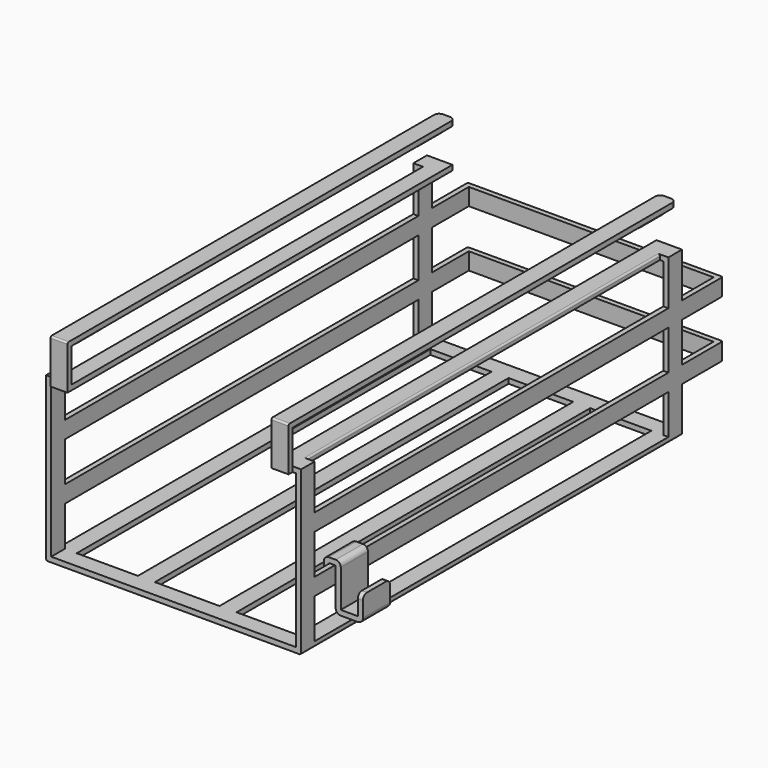
from build123d import *

# Parameters (mm, degrees)
F0_W           = 10
F0_H           = 260
F1_DEPTH       = 3
F2_W           = 3
F2_H           = 10
F3_DEPTH       = 90
F4_W           = 2
F4_H           = 10
F4_W_2         = 3
F4_W_3         = 10
F4_H_2         = 3
F4_W_4         = 5
F5_DEPTH       = 3
F6_W           = 10
F6_H           = 3
F7_DEPTH       = 20
F8_W           = 10
F8_H           = 282
F8_H_2         = 285
F8_H_3         = 3
F9_DEPTH       = 3
F10_W          = 3
F10_H          = 10
F11_DEPTH      = 30
F11_DEPTH_BACK = 270
F12_W          = 3
F12_H          = 10
F13_DEPTH      = 144
F14_R          = 1
F15_R          = 3
F17_DEPTH      = 1
F18_W          = 3
F18_H          = 20
F19_DEPTH      = 10
F18_W_2        = 0.5
F20_DEPTH      = 3
F21_DEPTH      = 25
F22_W          = 20
F22_H          = 3
F23_DEPTH      = 10
F24_W          = 3
F24_H          = 20
F25_DEPTH      = 15
F26_R          = 3


# Not quite as in the source:
# - a feature names something its author has since deleted; it is built from what else it names


with BuildPart() as f1:
    # F0 (on Top) → F1 (new body)
    with BuildSketch(Plane.XY):
        Polygon((-5.2808651924, 185.6500792865), (-155.2808651924, 185.6500792865), (-155.2808651924, 175.6500792865), (-145.2808651924, 175.6500792865), (-109.2808651924, 175.6500792865), (-99.2808651924, 175.6500792865), (-61.2808651924, 175.6500792865), (-51.2808651924, 175.6500792865), (-15.2808651924, 175.6500792865), (-5.2808651924, 175.6500792865), align=None)
        with Locations((-104.2808651924, 45.6500792865)):
            Rectangle(F0_W, F0_H)
        with Locations((-56.2808651924, 45.6500792865)):
            Rectangle(F0_W, F0_H)
        Polygon((-145.2808651924, -84.3499207135), (-155.2808651924, -84.3499207135), (-155.2808651924, -94.3499207135), (-5.2808651924, -94.3499207135), (-5.2808651924, -84.3499207135), (-15.2808651924, -84.3499207135), (-51.2808651924, -84.3499207135), (-61.2808651924, -84.3499207135), (-99.2808651924, -84.3499207135), (-109.2808651924, -84.3499207135), align=None)
        with Locations((-150.2808651924, 45.6500792865)):
            Rectangle(F0_W, F0_H)
        with Locations((-10.2808651924, 45.6500792865)):
            Rectangle(F0_W, F0_H)
    extrude(amount=F1_DEPTH)

    # F2 (on face) → F3 (join)
    with BuildSketch(Plane.XY.offset(3)):
        with Locations((-153.7808651924, 180.6500792865)):
            Rectangle(F2_W, F2_H)
        with Locations((-6.7808651924, 180.6500792865)):
            Rectangle(F2_W, F2_H)
        with Locations((-6.7808651924, -89.3499207135)):
            Rectangle(F2_W, F2_H)
        with Locations((-153.7808651924, -89.3499207135)):
            Rectangle(F2_W, F2_H)
    extrude(amount=F3_DEPTH)

    # F4 (on face) → F5 (join)
    with BuildSketch(Plane.XY.offset(93)):
        Polygon((-140.2808651924, 185.6500792865), (-150.2808651924, 185.6500792865), (-150.2808651924, 175.6500792865), (-150.2808651924, -84.3499207135), (-150.2808651924, -94.3499207135), (-140.2808651924, -94.3499207135), align=None)
        with Locations((-151.2808651924, 180.6500792865)):
            Rectangle(F4_W, F4_H)
        with Locations((-153.7808651924, 180.6500792865)):
            Rectangle(F4_W_2, F4_H)
        with Locations((-145.2808651924, -95.8499207135)):
            Rectangle(F4_W_3, F4_H_2)
        with Locations((-15.2808651924, -95.8499207135)):
            Rectangle(F4_W_3, F4_H_2)
        Polygon((-10.2808651924, 185.6500792865), (-20.2808651924, 185.6500792865), (-20.2808651924, -94.3499207135), (-10.2808651924, -94.3499207135), (-10.2808651924, -84.3499207135), (-10.2808651924, 175.6500792865), align=None)
        with Locations((-7.7808651924, -89.3499207135)):
            Rectangle(F4_W_4, F4_H)
        with Locations((-7.7808651924, 180.6500792865)):
            Rectangle(F4_W_4, F4_H)
        with Locations((-152.7808651924, -89.3499207135)):
            Rectangle(F4_W_4, F4_H)
    extrude(amount=F5_DEPTH)

    # F6 (on face) → F7 (join)
    with BuildSketch(Plane.XY.offset(96)):
        with Locations((-145.2808651924, -95.8499207135)):
            Rectangle(F6_W, F6_H)
        with Locations((-15.2808651924, -95.8499207135)):
            Rectangle(F6_W, F6_H)
    extrude(amount=F7_DEPTH)

    # F8 (on face) → F9 (join)
    with BuildSketch(Plane.XY.offset(116)):
        with Locations((-145.2808651924, 46.6500792865)):
            Rectangle(F8_W, F8_H)
        with Locations((-15.2808651924, 45.1500792865)):
            Rectangle(F8_W, F8_H_2)
        with Locations((-145.2808651924, -95.8499207135)):
            Rectangle(F8_W, F8_H_3)
    extrude(amount=F9_DEPTH)

    # F10 (on face) → F11 (join, two sides)
    with BuildSketch(Plane(origin=(0, 185.6500792865, 0), x_dir=(-1, 0, 0), z_dir=(0, 1, 0))) as f11_sk:
        with Locations((153.7808651924, 64.6666666667)):
            Rectangle(F10_W, F10_H)
        with Locations((153.7808651924, 31.3333333333)):
            Rectangle(F10_W, F10_H)
        with Locations((6.7808651924, 64.6666666667)):
            Rectangle(F10_W, F10_H)
        with Locations((6.7808651924, 31.3333333333)):
            Rectangle(F10_W, F10_H)
    extrude(amount=F11_DEPTH)
    extrude(f11_sk.sketch, amount=-F11_DEPTH_BACK)

    # F12 (on face) → F13 (join, through all)
    with BuildSketch(Plane.YZ.offset(-152.2808651924)):
        with Locations((214.1500792864, 64.6666666667)):
            Rectangle(F12_W, F12_H)
        with Locations((214.1500792864, 31.3333333333)):
            Rectangle(F12_W, F12_H)
    extrude(amount=F13_DEPTH)

    # F14
    f14_edges = [f1.edges().sort_by_distance(p)[0] for p in [
        (-155.280865, 45.650079, 0),
        (-5.280865, 45.650079, 0),
        (-5.280865, 215.650079, 31.333333),
        (-5.280865, 215.650079, 64.666667),
        (-155.280865, 215.650079, 64.666667),
        (-155.280865, 215.650079, 31.333333),
        (-150.280865, 45.650079, 96),
        (-145.280865, -97.349921, 119),
        (-15.280865, -97.349921, 119),
        (-10.280865, 45.650079, 96),
    ]]
    fillet(f14_edges, radius=F14_R)

    # F15
    f15_edges = [f1.edges().sort_by_distance(p)[0] for p in [
        (-140.280865, 187.650079, 117.5),
        (-150.280865, 187.650079, 117.5),
        (-20.280865, 187.650079, 117.5),
        (-10.280865, 187.650079, 117.5),
    ]]
    fillet(f15_edges, radius=F15_R)


with BuildPart() as f17:
    # F16 (on face) → F17 (new body)
    with BuildSketch(Plane(origin=(0, 0, 116), x_dir=(1, 0, 0), z_dir=(0, 0, -1))):
        with BuildLine():
            ThreePointArc((-149.3451507241, -179.0511412621), (-145.3451507241, -183.0511412621), (-141.3451507241, -179.0511412621))
            Line((-141.3451507241, -179.0511412621), (-141.3451507241, -162.0511412621))
            ThreePointArc((-141.3451507241, -162.0511412621), (-145.3451507241, -158.0511412621), (-149.3451507241, -162.0511412621))
            Line((-149.3451507241, -162.0511412621), (-149.3451507241, -179.0511412621))
        make_face()
    extrude(amount=F17_DEPTH)


with BuildPart() as f17b:
    # F16 (on face) → F17, piece 2 (new body)
    with BuildSketch(Plane(origin=(0, 0, 116), x_dir=(1, 0, 0), z_dir=(0, 0, -1))):
        with BuildLine():
            ThreePointArc((-11.2165796608, -162.0511412621), (-15.2165796608, -158.0511412621), (-19.2165796608, -162.0511412621))
            Line((-19.2165796608, -162.0511412621), (-19.2165796608, -179.0511412621))
            ThreePointArc((-19.2165796608, -179.0511412621), (-15.2165796608, -183.0511412621), (-11.2165796608, -179.0511412621))
            Line((-11.2165796608, -179.0511412621), (-11.2165796608, -162.0511412621))
        make_face()
    extrude(amount=F17_DEPTH)


with BuildPart() as f17c:
    # F16 (on face) → F17, piece 3 (new body)
    with BuildSketch(Plane(origin=(0, 0, 116), x_dir=(1, 0, 0), z_dir=(0, 0, -1))):
        with BuildLine():
            ThreePointArc((-11.2165796608, 88.7509826891), (-15.2165796608, 92.7509826891), (-19.2165796608, 88.7509826891))
            Line((-19.2165796608, 88.7509826891), (-19.2165796608, 71.7509826891))
            ThreePointArc((-19.2165796608, 71.7509826891), (-15.2165796608, 67.7509826891), (-11.2165796608, 71.7509826891))
            Line((-11.2165796608, 71.7509826891), (-11.2165796608, 88.7509826891))
        make_face()
    extrude(amount=F17_DEPTH)


with BuildPart() as f17d:
    # F16 (on face) → F17, piece 4 (new body)
    with BuildSketch(Plane(origin=(0, 0, 116), x_dir=(1, 0, 0), z_dir=(0, 0, -1))):
        with BuildLine():
            Line((-149.3451507241, 88.7509826891), (-149.3451507241, 71.7509826891))
            ThreePointArc((-149.3451507241, 71.7509826891), (-145.3451507241, 67.7509826891), (-141.3451507241, 71.7509826891))
            Line((-141.3451507241, 71.7509826891), (-141.3451507241, 88.7509826891))
            ThreePointArc((-141.3451507241, 88.7509826891), (-145.3451507241, 92.7509826891), (-149.3451507241, 88.7509826891))
        make_face()
    extrude(amount=F17_DEPTH)


with BuildPart() as f19:
    # F18 (on face) → F19 (new body, through all)
    with BuildSketch(Plane.XY.offset(36.3333333333)):
        with Locations((-10.2808651924, -59.5772841573)):
            Rectangle(F18_W, F18_H)
    extrude(amount=-F19_DEPTH)

    # F18 (on face) → F20 (join)
    with BuildSketch(Plane.XY.offset(36.3333333333)):
        with Locations((-10.2808651924, -59.5772841573)):
            Rectangle(F18_W, F18_H)
        with Locations((-6.7808651924, -59.5772841573)):
            Rectangle(F18_W, F18_H)
        with Locations((-8.5308651924, -59.5772841573)):
            Rectangle(F18_W_2, F18_H)
        with Locations((-5.0308651924, -59.5772841573)):
            Rectangle(F18_W_2, F18_H)
        with Locations((-3.2808651924, -59.5772841573)):
            Rectangle(F18_W, F18_H)
    extrude(amount=F20_DEPTH)

    # F18 (on face) → F21 (join)
    with BuildSketch(Plane.XY.offset(36.3333333333)):
        with Locations((-3.2808651924, -59.5772841573)):
            Rectangle(F18_W, F18_H)
    extrude(amount=-F21_DEPTH)

    # F22 (on face) → F23 (join)
    with BuildSketch(Plane.YZ.offset(-1.7808651924)):
        with Locations((-59.5772841573, 12.8333333333)):
            Rectangle(F22_W, F22_H)
    extrude(amount=F23_DEPTH)

    # F24 (on face) → F25 (join)
    with BuildSketch(Plane(origin=(0, 0, 11.3333333333), x_dir=(1, 0, 0), z_dir=(0, 0, -1))):
        with Locations((9.7191348076, 59.5772841573)):
            Rectangle(F24_W, F24_H)
    extrude(amount=-F25_DEPTH)

    # F26
    f26_edges = [f19.edges().sort_by_distance(p)[0] for p in [
        (9.719135, -69.577284, 26.333333),
        (9.719135, -49.577284, 26.333333),
        (11.219135, -59.577284, 11.333333),
        (-4.780865, -59.577284, 11.333333),
        (-1.780865, -59.577284, 39.333333),
        (-11.780865, -59.577284, 39.333333),
        (-10.280865, -69.577284, 26.333333),
        (-10.280865, -49.577284, 26.333333),
    ]]
    fillet(f26_edges, radius=F26_R)


solid = Compound([f1.part, f17.part, f17b.part, f17c.part, f17d.part, f19.part])
